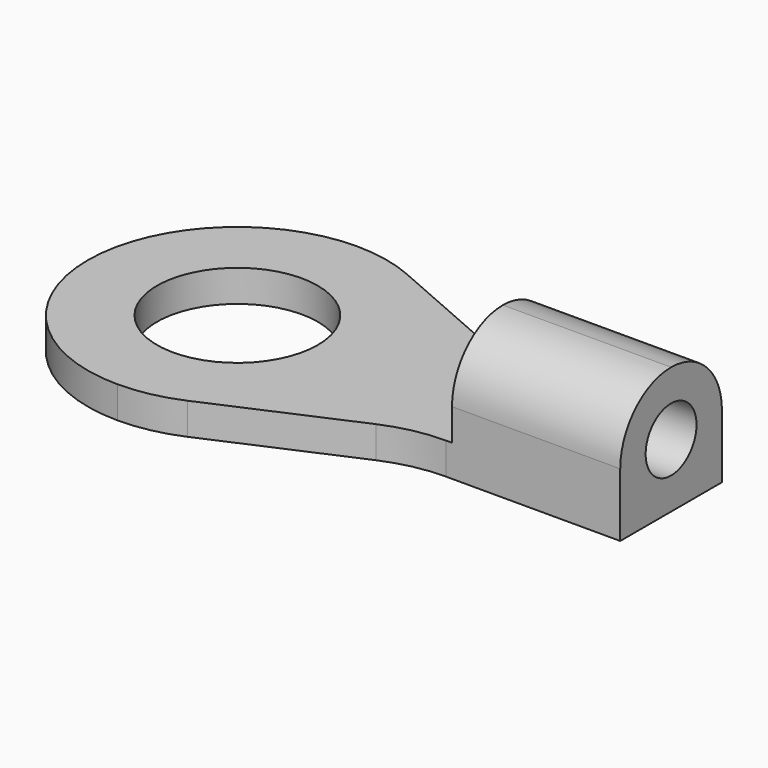
from build123d import *

# Parameters (mm, degrees)
F0_R     = 2.15
F1_DEPTH = 0.85
F2_W     = 4.5
F2_H     = 3.4
F3_DEPTH = 2.55
F4_R     = 1.69999
F5_R     = 0.85
F6_DEPTH = 25


# Not quite as in the source:
# - a fillet or chamfer is up to 0.001 mm smaller than in the source, because OpenCascade refuses the exact size


with BuildPart() as f1:
    # F0 (on Top) → F1 (new body)
    with BuildSketch(Plane.XY):
        with BuildLine():
            Line((10.9356666081, 2.3), (15.6, 2.3))
            Line((15.6, 2.3), (15.6, 5.7))
            Line((15.6, 5.7), (10.9356666081, 5.7))
            ThreePointArc((10.9356666081, 5.7), (10.117660762, 5.7845349656), (9.3342299639, 6.0345667821))
            Line((9.3342299639, 6.0345667821), (5.6014366442, 7.6654332179))
            ThreePointArc((5.6014366442, 7.6654332179), (4.8180058461, 7.9154650344), (4, 8))
            ThreePointArc((4, 8), (1.1715728753, 6.8284271247), (0, 4))
            ThreePointArc((0, 4), (1.1715728753, 1.1715728753), (4, 0))
            ThreePointArc((4, 0), (4.8180058461, 0.0845349656), (5.6014366442, 0.3345667821))
            Line((5.6014366442, 0.3345667821), (9.3342299639, 1.9654332179))
            ThreePointArc((9.3342299639, 1.9654332179), (10.117660762, 2.2154650344), (10.9356666081, 2.3))
        make_face()
        with Locations((4, 4)):
            Circle(F0_R, mode=Mode.SUBTRACT)
    extrude(amount=F1_DEPTH)

    # F2 (on face) → F3 (join)
    with BuildSketch(Plane.XY.offset(0.85)):
        with Locations((13.35, 4)):
            Rectangle(F2_W, F2_H)
    extrude(amount=F3_DEPTH)

    # F4 (radius 1.7 in the source; OpenCascade refuses exactly that, so slightly less here)
    f4_edges = [f1.edges().sort_by_distance(p)[0] for p in [
        (13.35, 5.7, 3.4),
        (13.35, 2.3, 3.4),
    ]]
    fillet(f4_edges, radius=F4_R)

    # F5 (on face) → F6 (cut)
    with BuildSketch(Plane.YZ.offset(15.6)):
        with Locations((4, 1.7)):
            Circle(F5_R)
    extrude(amount=-F6_DEPTH, mode=Mode.SUBTRACT)


solid = f1.part
